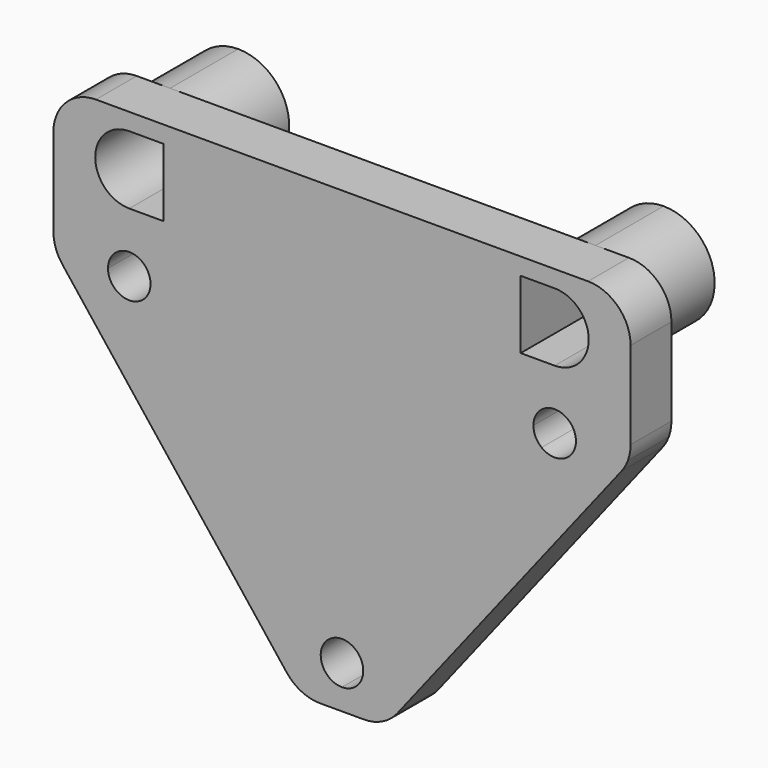
from build123d import *

# Parameters (mm, degrees)
F1_DEPTH = 6
F3_DEPTH = 10


with BuildPart() as f1:
    # F0 (on Front) → F1 (new body)
    with BuildSketch(Plane.XZ):
        with BuildLine():
            Line((-22.5, 14.5380757153), (-15.95, 14.5380757153))
            Line((-15.95, 14.5380757153), (15.95, 14.5380757153))
            Line((15.95, 14.5380757153), (22.5, 14.5380757153))
            ThreePointArc((22.5, 14.5380757153), (25, 17.0380757153), (27.5, 14.5380757153))
            Line((27.5, 14.5380757153), (33.6112053721, 14.5380757153))
            ThreePointArc((33.6112053721, 14.5380757153), (33.8410734014, 15.3874164322), (33.9184952978, 16.2639007813))
            Line((33.9184952978, 16.2639007813), (33.9184952978, 19.5380757153))
            Line((33.9184952978, 19.5380757153), (25, 19.5380757153))
            Line((25, 19.5380757153), (-25, 19.5380757153))
            Line((-25, 19.5380757153), (-33.9184952978, 19.5380757153))
            Line((-33.9184952978, 19.5380757153), (-33.9184952978, 16.2639007813))
            ThreePointArc((-33.9184952978, 16.2639007813), (-33.8410734014, 15.3874164322), (-33.6112053721, 14.5380757153))
            Line((-33.6112053721, 14.5380757153), (-27.5, 14.5380757153))
            ThreePointArc((-27.5, 14.5380757153), (-25, 17.0380757153), (-22.5, 14.5380757153))
        make_face()
        with BuildLine():
            Line((15.95, 14.5380757153), (-15.95, 14.5380757153))
            Line((-15.95, 14.5380757153), (-22.5, 14.5380757153))
            ThreePointArc((-22.5, 14.5380757153), (-22.7521952698, 13.4438299043), (-23.457899116, 12.5703549873))
            Line((-23.457899116, 12.5703549873), (-1.542100884, -15.3942035567))
            ThreePointArc((-1.542100884, -15.3942035567), (0, -14.8619242847), (1.542100884, -15.3942035567))
            Line((1.542100884, -15.3942035567), (23.457899116, 12.5703549873))
            ThreePointArc((23.457899116, 12.5703549873), (22.7521952698, 13.4438299043), (22.5, 14.5380757153))
            Line((22.5, 14.5380757153), (15.95, 14.5380757153))
        make_face()
        with BuildLine():
            ThreePointArc((-23.457899116, 12.5703549873), (-26.094245811, 12.2902709851), (-27.5, 14.5380757153))
            Line((-27.5, 14.5380757153), (-33.6112053721, 14.5380757153))
            ThreePointArc((-33.6112053721, 14.5380757153), (-33.28570797, 13.8292645711), (-32.8539367538, 13.1796990132))
            Line((-32.8539367538, 13.1796990132), (-6.5014092727, -20.4461260528))
            ThreePointArc((-6.5014092727, -20.4461260528), (-4.7544594387, -21.8575337451), (-2.5659678166, -22.3619242847))
            Line((-2.5659678166, -22.3619242847), (0, -22.3619242847))
            Line((0, -22.3619242847), (0, -19.8619242847))
            ThreePointArc((0, -19.8619242847), (-2.3631866008, -18.1776136189), (-1.542100884, -15.3942035567))
            Line((-1.542100884, -15.3942035567), (-23.457899116, 12.5703549873))
        make_face()
        with BuildLine():
            Line((33.6112053721, 14.5380757153), (27.5, 14.5380757153))
            ThreePointArc((27.5, 14.5380757153), (26.094245811, 12.2902709851), (23.457899116, 12.5703549873))
            Line((23.457899116, 12.5703549873), (1.542100884, -15.3942035567))
            ThreePointArc((1.542100884, -15.3942035567), (2.2478047302, -16.2676784737), (2.5, -17.3619242847))
            ThreePointArc((2.5, -17.3619242847), (1.767766953, -19.1296912377), (0, -19.8619242847))
            Line((0, -19.8619242847), (0, -22.3619242847))
            Line((0, -22.3619242847), (2.5659678166, -22.3619242847))
            ThreePointArc((2.5659678166, -22.3619242847), (4.7544594387, -21.8575337451), (6.5014092727, -20.4461260528))
            Line((6.5014092727, -20.4461260528), (32.8539367538, 13.1796990132))
            ThreePointArc((32.8539367538, 13.1796990132), (33.28570797, 13.8292645711), (33.6112053721, 14.5380757153))
        make_face()
        with BuildLine():
            Line((-33.9184952978, 26.5380757153), (-33.9184952978, 19.5380757153))
            Line((-33.9184952978, 19.5380757153), (-25, 19.5380757153))
            Line((-25, 19.5380757153), (-25, 21.5380757153))
            ThreePointArc((-25, 21.5380757153), (-29, 25.5380757153), (-25, 29.5380757153))
            Line((-25, 29.5380757153), (-25, 31.5380757153))
            Line((-25, 31.5380757153), (-28.9184952978, 31.5380757153))
            ThreePointArc((-28.9184952978, 31.5380757153), (-32.4540292037, 30.0736096212), (-33.9184952978, 26.5380757153))
        make_face()
        with BuildLine():
            Line((25, 19.5380757153), (33.9184952978, 19.5380757153))
            Line((33.9184952978, 19.5380757153), (33.9184952978, 26.5380757153))
            ThreePointArc((33.9184952978, 26.5380757153), (32.4540292037, 30.0736096212), (28.9184952978, 31.5380757153))
            Line((28.9184952978, 31.5380757153), (25, 31.5380757153))
            Line((25, 31.5380757153), (25, 29.5380757153))
            ThreePointArc((25, 29.5380757153), (27.8284271247, 28.36650284), (29, 25.5380757153))
            ThreePointArc((29, 25.5380757153), (27.8284271247, 22.7096485906), (25, 21.5380757153))
            Line((25, 21.5380757153), (25, 19.5380757153))
        make_face()
        Polygon((-25, 21.5380757153), (-25, 19.5380757153), (25, 19.5380757153), (25, 21.5380757153), (21, 21.5380757153), (21, 25.5380757153), (21, 29.5380757153), (25, 29.5380757153), (25, 31.5380757153), (-25, 31.5380757153), (-25, 29.5380757153), (-21, 29.5380757153), (-21, 25.5380757153), (-21, 21.5380757153), align=None)
    extrude(amount=F1_DEPTH)

    # F2 (on face) → F3 (join)
    with BuildSketch(Plane(origin=(0, 0, 0), x_dir=(-1, 0, 0), z_dir=(0, 1, 0))):
        with BuildLine():
            ThreePointArc((-25, 31.5380757153), (-29.2426406871, 21.2954350282), (-19, 25.5380757153))
            ThreePointArc((-19, 25.5380757153), (-20.7573593129, 29.7807164024), (-25, 31.5380757153))
        make_face()
        with BuildLine():
            Line((-21, 29.5380757153), (-21, 21.5380757153))
            Line((-21, 21.5380757153), (-25, 21.5380757153))
            ThreePointArc((-25, 21.5380757153), (-29, 25.5380757153), (-25, 29.5380757153))
            Line((-25, 29.5380757153), (-21, 29.5380757153))
        make_face(mode=Mode.SUBTRACT)
        with BuildLine():
            ThreePointArc((31, 25.5380757153), (29.2426406871, 29.7807164024), (25, 31.5380757153))
            ThreePointArc((25, 31.5380757153), (20.7573593129, 21.2954350282), (31, 25.5380757153))
        make_face()
        with BuildLine():
            Line((21, 29.5380757153), (25, 29.5380757153))
            ThreePointArc((25, 29.5380757153), (29, 25.5380757153), (25, 21.5380757153))
            Line((25, 21.5380757153), (21, 21.5380757153))
            Line((21, 21.5380757153), (21, 29.5380757153))
        make_face(mode=Mode.SUBTRACT)
    extrude(amount=F3_DEPTH)


solid = f1.part
